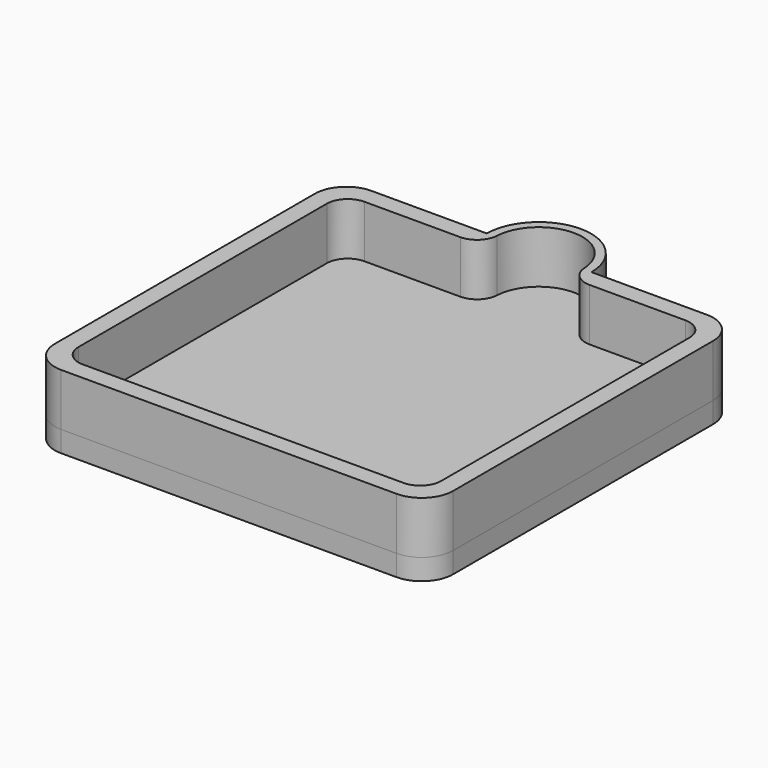
from build123d import *

# Parameters (mm, degrees)
F1_DEPTH = 2
F2_DEPTH = 5
F4_R     = 3
F4_2_R   = 3
F5_DEPTH = 5
F6_R     = 2
F7_R     = 2


with BuildPart() as f1:
    # F0 (on Top) → F1 (new body)
    with BuildSketch(Plane.XY):
        with BuildLine():
            Line((16, 15.5), (16, -15.5))
            Line((16, -15.5), (-16, -15.5))
            Line((-16, -15.5), (-16, 15.5))
            Line((-16, 15.5), (-4.0370162249, 15.5))
            ThreePointArc((-4.0370162249, 15.5), (-4.7608597882, 16.9221865044), (-4.9997499937, 18.5))
            Line((-4.9997499937, 18.5), (-19, 18.5))
            Line((-19, 18.5), (-19, -18.5))
            Line((-19, -18.5), (19, -18.5))
            Line((19, -18.5), (19, 18.5))
            Line((19, 18.5), (4.9997499937, 18.5))
            ThreePointArc((4.9997499937, 18.5), (4.999937498, 18.4750003125), (5, 18.45))
            ThreePointArc((5, 18.45), (4.7531611126, 16.8984010061), (4.0370162249, 15.5))
            Line((4.0370162249, 15.5), (16, 15.5))
        make_face()
        with BuildLine():
            Line((-16, -15.5), (16, -15.5))
            Line((16, -15.5), (16, 15.5))
            Line((16, 15.5), (4.0370162249, 15.5))
            ThreePointArc((4.0370162249, 15.5), (0, 13.45), (-4.0370162249, 15.5))
            Line((-4.0370162249, 15.5), (-16, 15.5))
            Line((-16, 15.5), (-16, -15.5))
        make_face()
        with BuildLine():
            ThreePointArc((-4.0370162249, 15.5), (0, 13.45), (4.0370162249, 15.5))
            Line((4.0370162249, 15.5), (1.6395502432, 15.5))
            ThreePointArc((1.6395502432, 15.5), (0, 15.075), (-1.6395502432, 15.5))
            Line((-1.6395502432, 15.5), (-4.0370162249, 15.5))
        make_face()
        with BuildLine():
            Line((1.6395502432, 15.5), (4.0370162249, 15.5))
            ThreePointArc((4.0370162249, 15.5), (4.7531611126, 16.8984010061), (5, 18.45))
            ThreePointArc((5, 18.45), (4.999937498, 18.4750003125), (4.9997499937, 18.5))
            Line((4.9997499937, 18.5), (3.3746296093, 18.5))
            ThreePointArc((3.3746296093, 18.5), (3.3749074011, 18.4750006859), (3.375, 18.45))
            ThreePointArc((3.375, 18.45), (2.908960903, 16.7386930537), (1.6395502432, 15.5))
        make_face()
        with BuildLine():
            ThreePointArc((-4.9997499937, 18.5), (-4.7608597882, 16.9221865044), (-4.0370162249, 15.5))
            Line((-4.0370162249, 15.5), (-1.6395502432, 15.5))
            ThreePointArc((-1.6395502432, 15.5), (-2.9215577862, 16.7602884561), (-3.3746296093, 18.5))
            Line((-3.3746296093, 18.5), (-4.9997499937, 18.5))
        make_face()
        with BuildLine():
            ThreePointArc((-1.6395502432, 15.5), (0, 15.075), (1.6395502432, 15.5))
            Line((1.6395502432, 15.5), (-1.6395502432, 15.5))
        make_face()
        with BuildLine():
            Line((-1.6395502432, 15.5), (1.6395502432, 15.5))
            ThreePointArc((1.6395502432, 15.5), (2.908960903, 16.7386930537), (3.375, 18.45))
            ThreePointArc((3.375, 18.45), (3.3749074011, 18.4750006859), (3.3746296093, 18.5))
            Line((3.3746296093, 18.5), (-3.3746296093, 18.5))
            ThreePointArc((-3.3746296093, 18.5), (-2.9215577862, 16.7602884561), (-1.6395502432, 15.5))
        make_face()
        with BuildLine():
            ThreePointArc((4.9997499937, 18.5), (0, 23.45), (-4.9997499937, 18.5))
            Line((-4.9997499937, 18.5), (-3.3746296093, 18.5))
            ThreePointArc((-3.3746296093, 18.5), (0, 21.825), (3.3746296093, 18.5))
            Line((3.3746296093, 18.5), (4.9997499937, 18.5))
        make_face()
        with BuildLine():
            ThreePointArc((3.3746296093, 18.5), (0, 21.825), (-3.3746296093, 18.5))
            Line((-3.3746296093, 18.5), (3.3746296093, 18.5))
        make_face()
    extrude(amount=-F1_DEPTH)

    # F4
    f4_edges = [f1.edges().sort_by_distance(p)[0] for p in [
        (-19, -18.5, -1),
        (19, -18.5, -1),
        (19, 18.5, -1),
        (-19, 18.5, -1),
    ]]
    fillet(f4_edges, radius=F4_R)


with BuildPart() as f2:
    # F0 (on Top) → F2 (new body)
    with BuildSketch(Plane.XY):
        with BuildLine():
            ThreePointArc((4.9997499937, 18.5), (0, 23.45), (-4.9997499937, 18.5))
            Line((-4.9997499937, 18.5), (-3.3746296093, 18.5))
            ThreePointArc((-3.3746296093, 18.5), (0, 21.825), (3.3746296093, 18.5))
            Line((3.3746296093, 18.5), (4.9997499937, 18.5))
        make_face()
        with BuildLine():
            Line((16, 15.5), (16, -15.5))
            Line((16, -15.5), (-16, -15.5))
            Line((-16, -15.5), (-16, 15.5))
            Line((-16, 15.5), (-4.0370162249, 15.5))
            ThreePointArc((-4.0370162249, 15.5), (-4.7608597882, 16.9221865044), (-4.9997499937, 18.5))
            Line((-4.9997499937, 18.5), (-19, 18.5))
            Line((-19, 18.5), (-19, -18.5))
            Line((-19, -18.5), (19, -18.5))
            Line((19, -18.5), (19, 18.5))
            Line((19, 18.5), (4.9997499937, 18.5))
            ThreePointArc((4.9997499937, 18.5), (4.999937498, 18.4750003125), (5, 18.45))
            ThreePointArc((5, 18.45), (4.7531611126, 16.8984010061), (4.0370162249, 15.5))
            Line((4.0370162249, 15.5), (16, 15.5))
        make_face()
        with BuildLine():
            Line((1.6395502432, 15.5), (4.0370162249, 15.5))
            ThreePointArc((4.0370162249, 15.5), (4.7531611126, 16.8984010061), (5, 18.45))
            ThreePointArc((5, 18.45), (4.999937498, 18.4750003125), (4.9997499937, 18.5))
            Line((4.9997499937, 18.5), (3.3746296093, 18.5))
            ThreePointArc((3.3746296093, 18.5), (3.3749074011, 18.4750006859), (3.375, 18.45))
            ThreePointArc((3.375, 18.45), (2.908960903, 16.7386930537), (1.6395502432, 15.5))
        make_face()
        with BuildLine():
            ThreePointArc((-4.9997499937, 18.5), (-4.7608597882, 16.9221865044), (-4.0370162249, 15.5))
            Line((-4.0370162249, 15.5), (-1.6395502432, 15.5))
            ThreePointArc((-1.6395502432, 15.5), (-2.9215577862, 16.7602884561), (-3.3746296093, 18.5))
            Line((-3.3746296093, 18.5), (-4.9997499937, 18.5))
        make_face()
    extrude(amount=F2_DEPTH)

    # F4#2
    f4_2_edges = [f2.edges().sort_by_distance(p)[0] for p in [
        (19, 18.5, 2.5),
        (-19, 18.5, 2.5),
        (19, -18.5, 2.5),
        (-19, -18.5, 2.5),
    ]]
    fillet(f4_2_edges, radius=F4_2_R)

    # F3 (on face) → F5 (cut)
    with BuildSketch(Plane.XY.offset(5)):
        with BuildLine():
            Line((-17.3, -16.8), (17.3, -16.8))
            Line((17.3, -16.8), (17.3, 16.8))
            Line((17.3, 16.8), (3.8351173385, 16.8))
            ThreePointArc((3.8351173385, 16.8), (0, 14.275), (-3.8351173385, 16.8))
            Line((-3.8351173385, 16.8), (-17.3, 16.8))
            Line((-17.3, 16.8), (-17.3, -16.8))
        make_face()
        with BuildLine():
            ThreePointArc((-3.8351173385, 16.8), (0, 14.275), (3.8351173385, 16.8))
            Line((3.8351173385, 16.8), (-3.8351173385, 16.8))
        make_face()
        with BuildLine():
            Line((-3.8351173385, 16.8), (3.8351173385, 16.8))
            ThreePointArc((3.8351173385, 16.8), (4.0891466034, 17.6076787692), (4.175, 18.45))
            ThreePointArc((4.175, 18.45), (-0.8423212308, 22.5391466034), (-3.8351173385, 16.8))
        make_face()
    extrude(amount=-F5_DEPTH, mode=Mode.SUBTRACT)

    # F6
    f6_edges = [f2.edges().sort_by_distance(p)[0] for p in [
        (-17.3, 16.8, 2.5),
        (17.3, 16.8, 2.5),
        (17.3, -16.8, 2.5),
        (-17.3, -16.8, 2.5),
    ]]
    fillet(f6_edges, radius=F6_R)

    # F7
    f7_edges = [f2.edges().sort_by_distance(p)[0] for p in [
        (-3.835117, 16.8, 2.5),
        (3.835117, 16.8, 2.5),
    ]]
    fillet(f7_edges, radius=F7_R)


solid = Compound([f1.part, f2.part])
